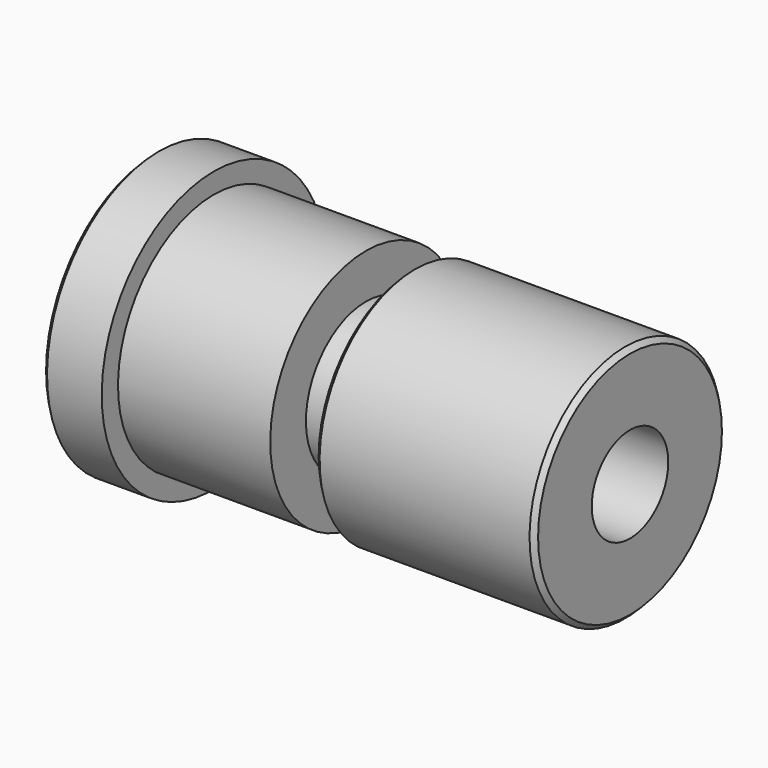
from build123d import *

# Parameters (mm, degrees)
F2_SIZE = 0.254
F4_D    = 5.1054


with BuildPart() as f1:
    # F0 (on Front) → F1 (revolve)
    with BuildSketch(Plane.XZ):
        Polygon((11.303, 6.3881), (3.175, 6.3881), (3.175, 7.47395), (0, 7.47395), (0, 0), (22.86, 0), (25.4, 0), (25.4, 6.3881), (13.68425, 6.3881), (13.68425, 4.00685), (11.303, 4.00685), align=None)
    revolve(axis=Axis((11.43, 0, 0), (1, 0, 0)))

    # F2
    f2_edges = [f1.edges().sort_by_distance(p)[0] for p in [
        (0, 0, -7.47395),
        (25.4, 0, -6.3881),
        (13.68425, 0, -6.3881),
    ]]
    chamfer(f2_edges, length=F2_SIZE)

    # F4 (through all)
    with Locations(Plane.YZ.offset(25.4)):
        with Locations((0, 0)):
            Hole(F4_D / 2)


solid = f1.part
